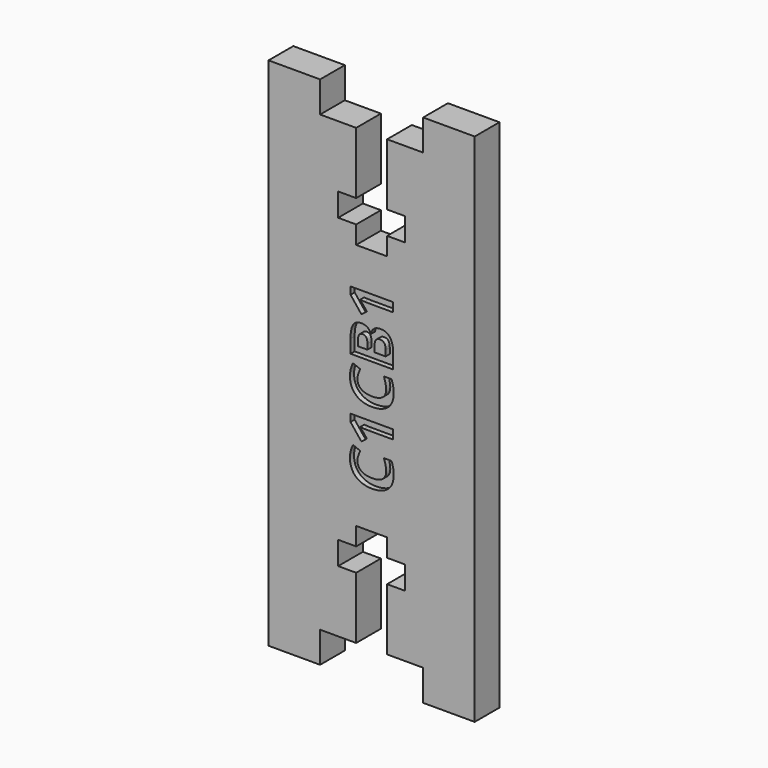
from build123d import *

# Parameters (mm, degrees)
F2_DEPTH     = 3
F5_TEXT_SIZE = 5.7808058854
F6_DEPTH     = 0.5


# Not quite as in the source:
# - Text() gives the source's letters only with a copy of the font that has no kerning and outlines rounded to 1/6400 em; it was checked with that copy


with BuildPart() as f2:
    # F1 (on Front) → F2 (new body)
    with BuildSketch(Plane.XZ):
        Polygon((-4.9999997765, 25), (-9.9999997765, 25), (-9.9999997765, 0), (2.235e-07, 0), (2.235e-07, 12), (-1.4999997765, 12), (-1.4999997765, 13.75), (-3.2499997765, 13.75), (-3.2499997765, 16), (-1.4999997765, 16), (-1.4999997765, 22), (-4.9999997765, 22), align=None)
    extrude(amount=F2_DEPTH)

    # F3: F2 across plane


with BuildPart() as f2_1:
    add(f2.part)
    add(f2.part.mirror(Plane.YZ))

    # F4: F2 across plane


with BuildPart() as f2_2:
    add(f2_1.part)
    add(f2_1.part.mirror(Plane.XY))

    # F5 (on face) → F6 (cut)
    with BuildSketch(Plane.XZ.offset(3)):
        with Locations(Location((2.0810901187, -8.6567568134), (0, 0, 90))):
            Text('C1CB1', F5_TEXT_SIZE, font='Open Sans', font_style=FontStyle.BOLD, text_align=(TextAlign.LEFT, TextAlign.BOTTOM))
    extrude(amount=-F6_DEPTH, mode=Mode.SUBTRACT)


solid = f2_2.part
